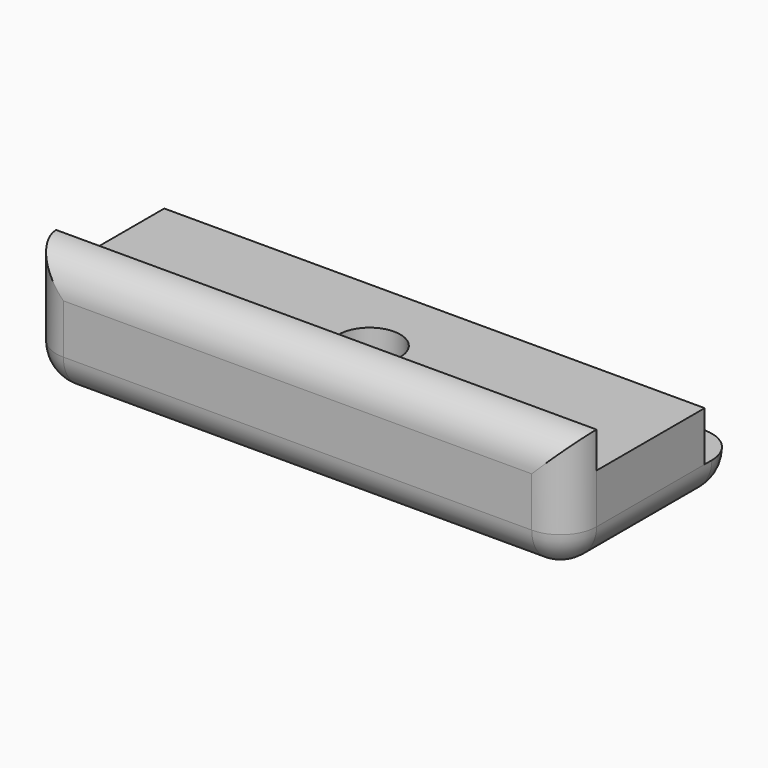
from build123d import *

# Parameters (mm, degrees)
F0_W     = 30
F0_H     = 2.5
F1_DEPTH = 2
F0_H_2   = 7.5
F0_R     = 1.7
F2_DEPTH = 4.75
F0_H_3   = 2
F3_DEPTH = 6.75
F4_R     = 1.99999


# Not quite as in the source:
# - a fillet or chamfer is up to 0.001 mm smaller than in the source, because OpenCascade refuses the exact size


with BuildPart() as f1:
    # F0 (on Top) → F1 (new body)
    with BuildSketch(Plane.XY):
        with Locations((7.8400733322, 0.8872417808)):
            Rectangle(F0_W, F0_H)
    extrude(amount=F1_DEPTH)

    # F0 (on Top) → F2 (join)
    with BuildSketch(Plane.XY):
        with Locations((7.8400733322, -4.1127582192)):
            Rectangle(F0_W, F0_H_2)
        with Locations((7.8400733322, -4.8627582192)):
            Circle(F0_R, mode=Mode.SUBTRACT)
    extrude(amount=F2_DEPTH)

    # F0 (on Top) → F3 (join)
    with BuildSketch(Plane.XY):
        with Locations((7.8400733322, -8.8627582192)):
            Rectangle(F0_W, F0_H_3)
    extrude(amount=F3_DEPTH)

    # F4 (radius 2 in the source; OpenCascade refuses exactly that, so slightly less here)
    f4_edges = [f1.edges().sort_by_distance(p)[0] for p in [
        (-7.159927, 2.137242, 1),
        (22.840073, 2.137242, 1),
        (-7.159927, -9.862758, 3.375),
        (22.840073, -9.862758, 3.375),
        (7.840073, 2.137242, 0),
        (22.840073, -3.862758, 0),
        (-7.159927, -3.862758, 0),
        (7.840073, -9.862758, 0),
        (7.840073, -9.862758, 6.75),
    ]]
    fillet(f4_edges, radius=F4_R)


solid = f1.part
